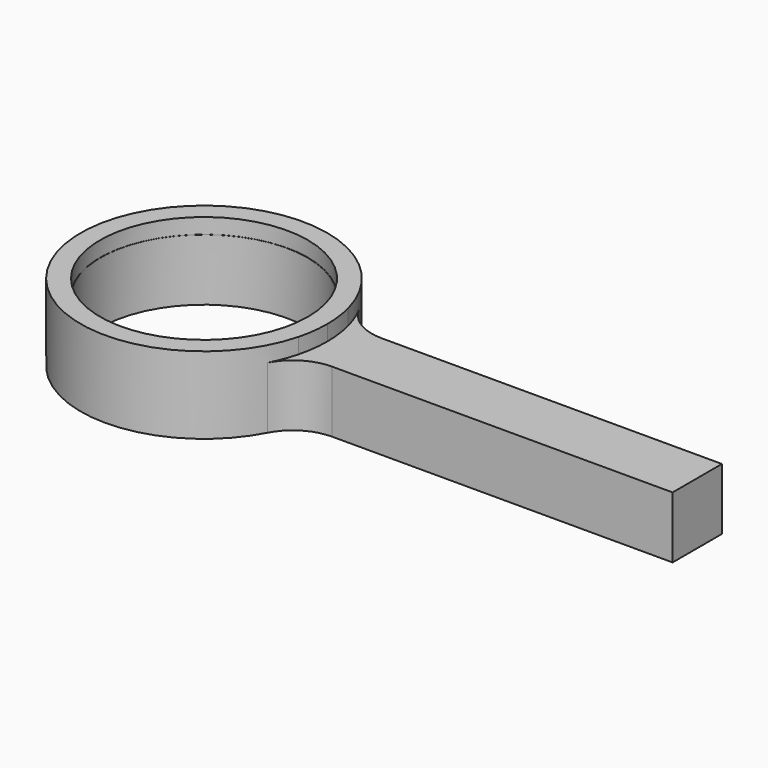
from build123d import *

# Parameters (mm, degrees)
F0_R        = 10.6794819522
F1_DEPTH    = 6.35
F2_R        = 10.6995432546
F3_DEPTH    = 1.5875
F4_T1_DEPTH = 6.35
F5_T1_DEPTH = 6.35


# Not quite as in the source:
# - a fillet or chamfer that OpenCascade refuses, or shapes differently, is made with other operations: its cross-section is extruded or revolved along the edge and cut away or added


with BuildPart() as f1:
    # F0 (on Top) → F1 (new body)
    with BuildSketch(Plane.XY):
        with BuildLine():
            Line((50.8, 3.175), (12.2967221242, 3.175))
            ThreePointArc((12.2967221242, 3.175), (-12.7, 0), (12.2967221242, -3.175))
            Line((12.2967221242, -3.175), (50.8, -3.175))
            Line((50.8, -3.175), (50.8, 3.175))
        make_face()
        Circle(F0_R, mode=Mode.SUBTRACT)
    extrude(amount=F1_DEPTH)

    # F2 (on face) → F3 (join)
    with BuildSketch(Plane.XY.offset(6.35)):
        with BuildLine():
            ThreePointArc((12.2967221242, -3.175), (12.5987771426, -1.6002545145), (12.7, 0))
            ThreePointArc((12.7, 0), (12.5987771426, 1.6002545145), (12.2967221242, 3.175))
            ThreePointArc((12.2967221242, 3.175), (-12.7, 0), (12.2967221242, -3.175))
        make_face()
        Circle(F2_R, mode=Mode.SUBTRACT)
    extrude(amount=F3_DEPTH)

    # F4: fillet of radius 5.08 on 1 edges, made by hand

    # F4_s2 → F4_t1 (join)
    with BuildSketch(Plane.XY):
        with BuildLine():
            ThreePointArc((15.7474878949, -3.175), (13.1183381138, -3.908280383), (11.2482056392, -5.8964285714))
            ThreePointArc((11.2482056392, -5.8964285714), (11.8508417091, -4.5659118242), (12.2967221242, -3.175))
            Line((12.2967221242, -3.175), (15.7474878949, -3.175))
        make_face()
    extrude(amount=F4_T1_DEPTH)

    # F5: fillet of radius 5.08 on 1 edges, made by hand

    # F5_s2 → F5_t1 (join)
    with BuildSketch(Plane.XY):
        with BuildLine():
            ThreePointArc((15.7474878949, 3.175), (13.1183381138, 3.908280383), (11.2482056392, 5.8964285714))
            ThreePointArc((11.2482056392, 5.8964285714), (11.8508417091, 4.5659118242), (12.2967221242, 3.175))
            Line((12.2967221242, 3.175), (15.7474878949, 3.175))
        make_face()
    extrude(amount=F5_T1_DEPTH)


solid = f1.part
